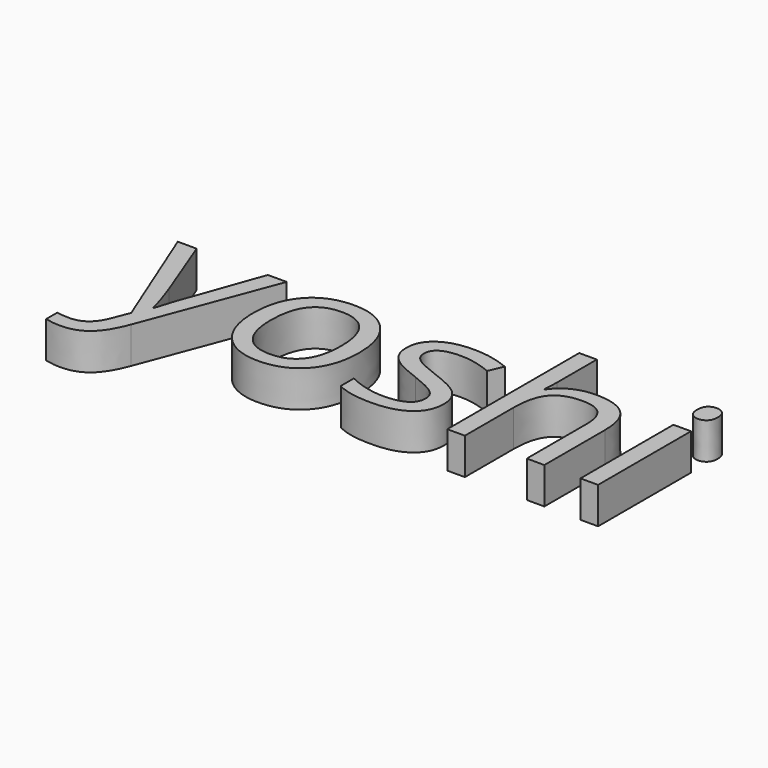
from build123d import *

# Parameters (mm, degrees)
F0_TEXT_SIZE = 151.0312728998
F1_DEPTH     = 25.4


# Not quite as in the source:
# - Text() gives the source's letters only with a copy of the font that has no kerning and outlines rounded to 1/6400 em; it was checked with that copy


with BuildPart() as f1:
    # F0 (on Top) → F1 (new body)
    with BuildSketch(Plane.XY):
        with Locations((-120.7512021065, -69.9373856187)):
            Text('yoshi', F0_TEXT_SIZE, font='Open Sans', text_align=(TextAlign.LEFT, TextAlign.BOTTOM))
    extrude(amount=F1_DEPTH)


solid = f1.part
